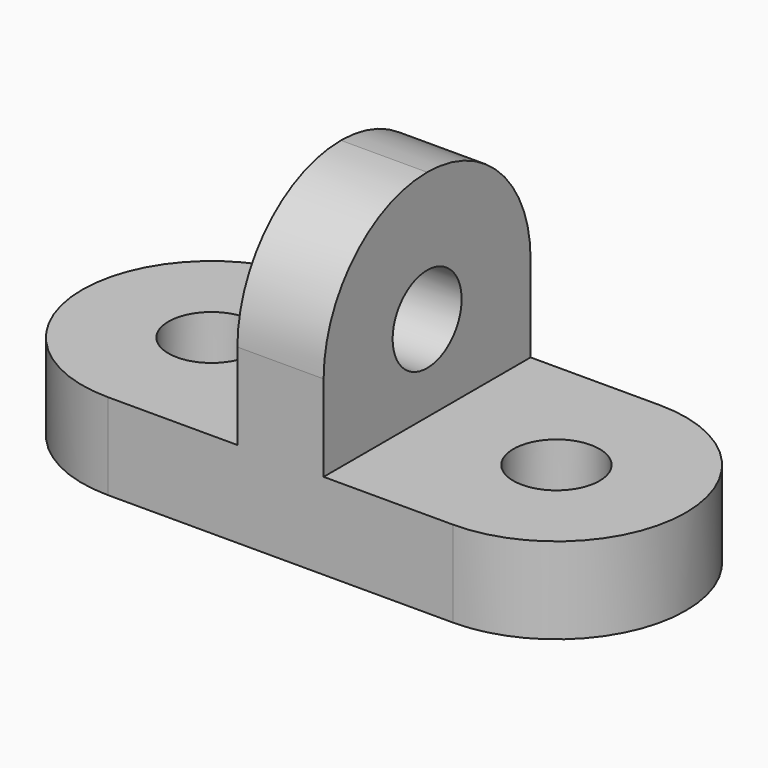
from build123d import *

# Parameters (mm, degrees)
F0_R     = 5
F0_W     = 10
F0_H     = 30
F1_DEPTH = 10
F2_DEPTH = 35
F3_R     = 14.99999
F5_D     = 10


# Not quite as in the source:
# - a fillet or chamfer is up to 0.001 mm smaller than in the source, because OpenCascade refuses the exact size


with BuildPart() as f1:
    # F0 (on Top) → F1 (new body)
    with BuildSketch(Plane.XY):
        with BuildLine():
            ThreePointArc((-20, 15), (-35, 0), (-20, -15))
            Line((-20, -15), (-5, -15))
            Line((-5, -15), (-5, 15))
            Line((-5, 15), (-20, 15))
        make_face()
        with Locations((-20, 0)):
            Circle(F0_R, mode=Mode.SUBTRACT)
        with BuildLine():
            Line((5, 15), (5, -15))
            Line((5, -15), (20, -15))
            ThreePointArc((20, -15), (35, 0), (20, 15))
            Line((20, 15), (5, 15))
        make_face()
        with Locations((20, 0)):
            Circle(F0_R, mode=Mode.SUBTRACT)
        Rectangle(F0_W, F0_H)
    extrude(amount=F1_DEPTH)

    # F0 (on Top) → F2 (join)
    with BuildSketch(Plane.XY):
        Rectangle(F0_W, F0_H)
    extrude(amount=F2_DEPTH)

    # F3 (radius 15 in the source; OpenCascade refuses exactly that, so slightly less here)
    f3_edges = [f1.edges().sort_by_distance(p)[0] for p in [
        (0, -15, 35),
        (0, 15, 35),
    ]]
    fillet(f3_edges, radius=F3_R)

    # F5 (through all)
    with Locations(Plane.YZ.offset(5)):
        with Locations((0, 20)):
            Hole(F5_D / 2)


solid = f1.part
